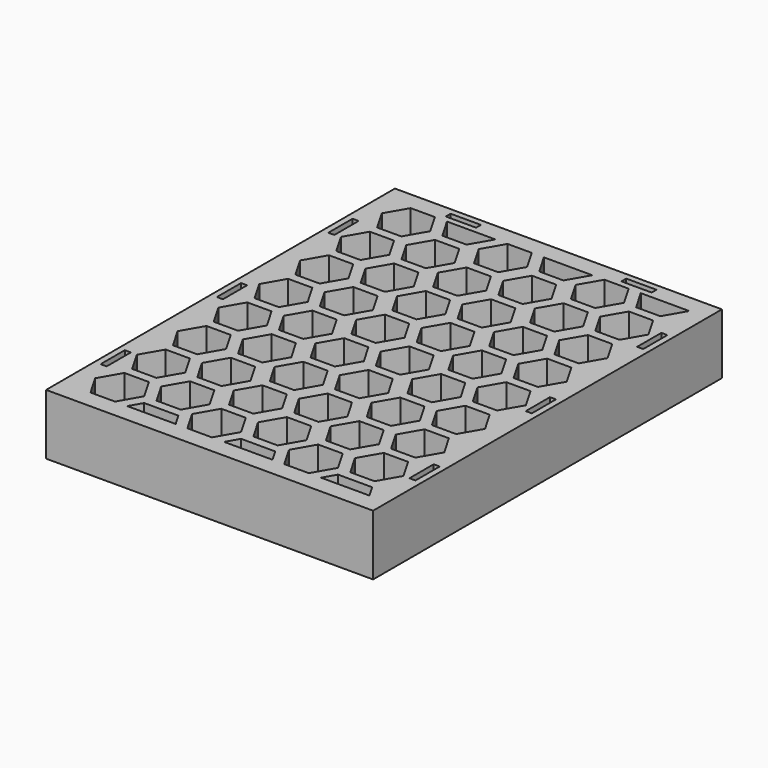
from build123d import *

# Parameters (mm, degrees)
F0_W     = 129.54
F0_H     = 179.07
F1_DEPTH = 25.4
F2_DEPTH = 25.4
F3_DEPTH = 25.4
F5_DEPTH = 25.4
F6_DEPTH = 25.4
F7_W     = 2.54
F7_H     = 12.7
F7_W_2   = 12.7
F7_H_2   = 2.54
F8_DEPTH = 7.62


# Not quite as in the source:
# - a feature names something its author has since deleted; it is built from what else it names


with BuildPart() as f1:
    # F0 (on Top) → F1 (new body)
    with BuildSketch(Plane.XY):
        with Locations((-8.2323685432, 21.6441547314)):
            Rectangle(F0_W, F0_H)
        Polygon((-69.4105034385, -51.3775724846), (-64.275970552, -42.4842987183), (-54.0069031043, -42.4842977514), (-48.8723685432, -51.3775705508), (-54.0069014297, -60.2708443171), (-64.2759688773, -60.270845284), align=None, mode=Mode.SUBTRACT)
        Polygon((-48.8723685432, -60.2708452686), (-45.8830056211, -55.0931168053), (-31.5417314652, -55.0931168053), (-28.5523685432, -60.2708452686), align=None, mode=Mode.SUBTRACT)
        Polygon((-28.7705034385, -51.3775720702), (-23.6359697633, -42.4842987593), (-13.3669023156, -42.4842987032), (-8.2323685432, -51.377571958), (-13.3669022184, -60.2708452689), (-23.635969666, -60.270845325), align=None, mode=Mode.SUBTRACT)
        Polygon((-48.8723685432, -42.4842987029), (-43.7923685432, -33.6854806004), (-33.6323685432, -33.6854806004), (-28.5523685432, -42.4842987029), (-33.6323685432, -51.2831168053), (-43.7923685432, -51.2831168053), align=None, mode=Mode.SUBTRACT)
        Polygon((-28.5523685432, -29.8754806837), (-23.4723685912, -21.0766625535), (-13.3123685912, -21.076662498), (-8.2323685432, -29.8754805727), (-13.3123684951, -38.6742987029), (-23.4723684951, -38.6742987584), align=None, mode=Mode.SUBTRACT)
        Polygon((-48.8723685432, -21.076662498), (-43.7923685432, -12.2778443955), (-33.6323685432, -12.2778443955), (-28.5523685432, -21.076662498), (-33.6323685432, -29.8754806004), (-43.7923685432, -29.8754806004), align=None, mode=Mode.SUBTRACT)
        Polygon((-48.8723685432, 0.3309737069), (-43.7923685432, 9.1297918094), (-33.6323685432, 9.1297918094), (-28.5523685432, 0.3309737069), (-33.6323685432, -8.4678443955), (-43.7923685432, -8.4678443955), align=None, mode=Mode.SUBTRACT)
        Polygon((-28.5523685432, -8.4678444788), (-23.4723685912, 0.3309736514), (-13.3123685912, 0.3309737069), (-8.2323685432, -8.4678443678), (-13.3123684951, -17.266662498), (-23.4723684951, -17.2666625535), align=None, mode=Mode.SUBTRACT)
        Polygon((-48.8723685432, 21.7386099118), (-43.7923685432, 30.5374280143), (-33.6323685432, 30.5374280143), (-28.5523685432, 21.7386099118), (-33.6323685432, 12.9397918094), (-43.7923685432, 12.9397918094), align=None, mode=Mode.SUBTRACT)
        Polygon((-28.5523685432, 12.9397917261), (-23.4723685912, 21.7386098563), (-13.3123685912, 21.7386099118), (-8.2323685432, 12.9397918371), (-13.3123684951, 4.1409737069), (-23.4723684951, 4.1409736514), align=None, mode=Mode.SUBTRACT)
        Polygon((-8.2323685432, -60.2708452686), (-5.2430056211, -55.0931168053), (9.0982685348, -55.0931168053), (12.0876314568, -60.2708452686), align=None, mode=Mode.SUBTRACT)
        Polygon((11.8694965615, -51.3775719857), (17.0040302854, -42.4842987029), (27.273097733, -42.4842987029), (32.4076314568, -51.3775719857), (27.273097733, -60.2708452686), (17.0040302854, -60.2708452686), align=None, mode=Mode.SUBTRACT)
        Polygon((-8.2323685432, -42.4842987029), (-3.1523685432, -33.6854806004), (7.0076314568, -33.6854806004), (12.0876314568, -42.4842987029), (7.0076314568, -51.2831168053), (-3.1523685432, -51.2831168053), align=None, mode=Mode.SUBTRACT)
        Polygon((12.0876314568, -29.8754806004), (17.1676314568, -21.076662498), (27.3276314568, -21.076662498), (32.4076314568, -29.8754806004), (27.3276314568, -38.6742987029), (17.1676314568, -38.6742987029), align=None, mode=Mode.SUBTRACT)
        Polygon((32.4076314568, -60.2708452686), (35.3969943789, -55.0931168053), (49.7382685348, -55.0931168053), (52.7276314568, -60.2708452686), align=None, mode=Mode.SUBTRACT)
        Polygon((-8.2323685432, -21.076662498), (-3.1523685432, -12.2778443955), (7.0076314568, -12.2778443955), (12.0876314568, -21.076662498), (7.0076314568, -29.8754806004), (-3.1523685432, -29.8754806004), align=None, mode=Mode.SUBTRACT)
        Polygon((-8.2323685432, 0.3309737069), (-3.1523685432, 9.1297918094), (7.0076314568, 9.1297918094), (12.0876314568, 0.3309737069), (7.0076314568, -8.4678443955), (-3.1523685432, -8.4678443955), align=None, mode=Mode.SUBTRACT)
        Polygon((12.0876314568, -8.4678443955), (17.1676314568, 0.3309737069), (27.3276314568, 0.3309737069), (32.4076314568, -8.4678443955), (27.3276314568, -17.266662498), (17.1676314568, -17.266662498), align=None, mode=Mode.SUBTRACT)
        Polygon((-8.2323685432, 21.7386099118), (-3.1523685432, 30.5374280143), (7.0076314568, 30.5374280143), (12.0876314568, 21.7386099118), (7.0076314568, 12.9397918094), (-3.1523685432, 12.9397918094), align=None, mode=Mode.SUBTRACT)
        Polygon((12.0876314568, 12.9397918094), (17.1676314568, 21.7386099118), (27.3276314568, 21.7386099118), (32.4076314568, 12.9397918094), (27.3276314568, 4.1409737069), (17.1676314568, 4.1409737069), align=None, mode=Mode.SUBTRACT)
        Polygon((-48.8723685432, 43.1462461167), (-43.7923685432, 51.9450642192), (-33.6323685432, 51.9450642192), (-28.5523685432, 43.1462461167), (-33.6323685432, 34.3474280143), (-43.7923685432, 34.3474280143), align=None, mode=Mode.SUBTRACT)
        Polygon((-28.5523685432, 34.347427931), (-23.4723685912, 43.1462460612), (-13.3123685912, 43.1462461167), (-8.2323685432, 34.347428042), (-13.3123684951, 25.5486099118), (-23.4723684951, 25.5486098563), align=None, mode=Mode.SUBTRACT)
        Polygon((-48.8723685432, 64.5538823216), (-43.7923685432, 73.3527004241), (-33.6323685432, 73.3527004241), (-28.5523685432, 64.5538823216), (-33.6323685432, 55.7550642192), (-43.7923685432, 55.7550642192), align=None, mode=Mode.SUBTRACT)
        Polygon((-28.5523685432, 55.7550641359), (-23.4723685912, 64.5538822661), (-13.3123685912, 64.5538823216), (-8.2323685432, 55.7550642469), (-13.3123684951, 46.9562461167), (-23.4723684951, 46.9562460612), align=None, mode=Mode.SUBTRACT)
        Polygon((-69.1923685432, 98.5703361507), (-64.1123693716, 107.3691547314), (-53.9523693716, 107.369155688), (-48.8723685432, 98.5703380639), (-53.9523677147, 89.7715194831), (-64.1123677147, 89.7715185265), align=None, mode=Mode.SUBTRACT)
        Polygon((-48.8723685432, 85.9615185265), (-43.7923685432, 94.760336629), (-33.6323685432, 94.760336629), (-28.5523685432, 85.9615185265), (-33.6323685432, 77.1627004241), (-43.7923685432, 77.1627004241), align=None, mode=Mode.SUBTRACT)
        Polygon((-28.5523685432, 77.1627003408), (-23.4723685912, 85.961518471), (-13.3123685912, 85.9615185265), (-8.2323685432, 77.1627004518), (-13.3123684951, 68.3638823216), (-23.4723684951, 68.3638822661), align=None, mode=Mode.SUBTRACT)
        Polygon((-43.7923685432, 98.570336629), (-48.8723685432, 107.3691547314), (-28.5523685432, 107.3691547314), (-33.6323685432, 98.570336629), align=None, mode=Mode.SUBTRACT)
        Polygon((-28.5523685432, 98.5703365457), (-23.4723685912, 107.3691546759), (-13.3123685912, 107.3691547314), (-8.2323685432, 98.5703366567), (-13.3123684951, 89.7715185265), (-23.4723684951, 89.771518471), align=None, mode=Mode.SUBTRACT)
        Polygon((-8.2323685432, 43.1462461167), (-3.1523685432, 51.9450642192), (7.0076314568, 51.9450642192), (12.0876314568, 43.1462461167), (7.0076314568, 34.3474280143), (-3.1523685432, 34.3474280143), align=None, mode=Mode.SUBTRACT)
        Polygon((12.0876314568, 34.3474280143), (17.1676314568, 43.1462461167), (27.3276314568, 43.1462461167), (32.4076314568, 34.3474280143), (27.3276314568, 25.5486099118), (17.1676314568, 25.5486099118), align=None, mode=Mode.SUBTRACT)
        Polygon((-8.2323685432, 64.5538823216), (-3.1523685432, 73.3527004241), (7.0076314568, 73.3527004241), (12.0876314568, 64.5538823216), (7.0076314568, 55.7550642192), (-3.1523685432, 55.7550642192), align=None, mode=Mode.SUBTRACT)
        Polygon((12.0876314568, 55.7550642192), (17.1676314568, 64.5538823216), (27.3276314568, 64.5538823216), (32.4076314568, 55.7550642192), (27.3276314568, 46.9562461167), (17.1676314568, 46.9562461167), align=None, mode=Mode.SUBTRACT)
        Polygon((-8.2323685432, 85.9615185265), (-3.1523685432, 94.760336629), (7.0076314568, 94.760336629), (12.0876314568, 85.9615185265), (7.0076314568, 77.1627004241), (-3.1523685432, 77.1627004241), align=None, mode=Mode.SUBTRACT)
        Polygon((12.0876314568, 77.1627004241), (17.1676314568, 85.9615185265), (27.3276314568, 85.9615185265), (32.4076314568, 77.1627004241), (27.3276314568, 68.3638823216), (17.1676314568, 68.3638823216), align=None, mode=Mode.SUBTRACT)
        Polygon((-3.1523685432, 98.570336629), (-8.2323685432, 107.3691547314), (12.0876314568, 107.3691547314), (7.0076314568, 98.570336629), align=None, mode=Mode.SUBTRACT)
        Polygon((12.0876314568, 98.570336629), (17.1676314568, 107.3691547314), (27.3276314568, 107.3691547314), (32.4076314568, 98.570336629), (27.3276314568, 89.7715185265), (17.1676314568, 89.7715185265), align=None, mode=Mode.SUBTRACT)
        Polygon((37.4876314568, 98.570336629), (32.4076314568, 107.3691547314), (52.7276314568, 107.3691547314), (47.6476314568, 98.570336629), align=None, mode=Mode.SUBTRACT)
        Polygon((27.273097733, -42.4842987029), (17.0040302854, -42.4842987029), (11.8694965615, -51.3775719857), (17.0040302854, -60.2708452686), (27.273097733, -60.2708452686), (32.4076314568, -51.3775719857), align=None)
        Polygon((-13.3669023156, -42.4842987032), (-23.6359697633, -42.4842987593), (-28.7705034385, -51.3775720702), (-23.635969666, -60.270845325), (-13.3669022184, -60.2708452689), (-8.2323685432, -51.377571958), align=None)
        Polygon((-54.0069031043, -42.4842977514), (-64.275970552, -42.4842987183), (-69.4105034385, -51.3775724846), (-64.2759688773, -60.270845284), (-54.0069014297, -60.2708443171), (-48.8723685432, -51.3775705508), align=None)
        Polygon((-33.6323685432, 51.9450642192), (-43.7923685432, 51.9450642192), (-48.8723685432, 43.1462461167), (-43.7923685432, 34.3474280143), (-33.6323685432, 34.3474280143), (-28.5523685432, 43.1462461167), align=None)
        Polygon((-13.3123685912, 43.1462461167), (-23.4723685912, 43.1462460612), (-28.5523685432, 34.347427931), (-23.4723684951, 25.5486098563), (-13.3123684951, 25.5486099118), (-8.2323685432, 34.347428042), align=None)
        Polygon((-13.3123685912, 21.7386099118), (-23.4723685912, 21.7386098563), (-28.5523685432, 12.9397917261), (-23.4723684951, 4.1409736514), (-13.3123684951, 4.1409737069), (-8.2323685432, 12.9397918371), align=None)
        Polygon((-13.3123685912, 0.3309737069), (-23.4723685912, 0.3309736514), (-28.5523685432, -8.4678444788), (-23.4723684951, -17.2666625535), (-13.3123684951, -17.266662498), (-8.2323685432, -8.4678443678), align=None)
        Polygon((-33.6323685432, -12.2778443955), (-43.7923685432, -12.2778443955), (-48.8723685432, -21.076662498), (-43.7923685432, -29.8754806004), (-33.6323685432, -29.8754806004), (-28.5523685432, -21.076662498), align=None)
        Polygon((-13.3123685912, -21.076662498), (-23.4723685912, -21.0766625535), (-28.5523685432, -29.8754806837), (-23.4723684951, -38.6742987584), (-13.3123684951, -38.6742987029), (-8.2323685432, -29.8754805727), align=None)
        Polygon((-33.6323685432, -33.6854806004), (-43.7923685432, -33.6854806004), (-48.8723685432, -42.4842987029), (-43.7923685432, -51.2831168053), (-33.6323685432, -51.2831168053), (-28.5523685432, -42.4842987029), align=None)
        Polygon((7.0076314568, -12.2778443955), (-3.1523685432, -12.2778443955), (-8.2323685432, -21.076662498), (-3.1523685432, -29.8754806004), (7.0076314568, -29.8754806004), (12.0876314568, -21.076662498), align=None)
        Polygon((7.0076314568, 9.1297918094), (-3.1523685432, 9.1297918094), (-8.2323685432, 0.3309737069), (-3.1523685432, -8.4678443955), (7.0076314568, -8.4678443955), (12.0876314568, 0.3309737069), align=None)
        Polygon((27.3276314568, 0.3309737069), (17.1676314568, 0.3309737069), (12.0876314568, -8.4678443955), (17.1676314568, -17.266662498), (27.3276314568, -17.266662498), (32.4076314568, -8.4678443955), align=None)
        Polygon((27.3276314568, -21.076662498), (17.1676314568, -21.076662498), (12.0876314568, -29.8754806004), (17.1676314568, -38.6742987029), (27.3276314568, -38.6742987029), (32.4076314568, -29.8754806004), align=None)
        Polygon((27.3276314568, 21.7386099118), (17.1676314568, 21.7386099118), (12.0876314568, 12.9397918094), (17.1676314568, 4.1409737069), (27.3276314568, 4.1409737069), (32.4076314568, 12.9397918094), align=None)
        Polygon((7.0076314568, 30.5374280143), (-3.1523685432, 30.5374280143), (-8.2323685432, 21.7386099118), (-3.1523685432, 12.9397918094), (7.0076314568, 12.9397918094), (12.0876314568, 21.7386099118), align=None)
        Polygon((27.3276314568, 43.1462461167), (17.1676314568, 43.1462461167), (12.0876314568, 34.3474280143), (17.1676314568, 25.5486099118), (27.3276314568, 25.5486099118), (32.4076314568, 34.3474280143), align=None)
        Polygon((7.0076314568, 51.9450642192), (-3.1523685432, 51.9450642192), (-8.2323685432, 43.1462461167), (-3.1523685432, 34.3474280143), (7.0076314568, 34.3474280143), (12.0876314568, 43.1462461167), align=None)
        Polygon((27.3276314568, 64.5538823216), (17.1676314568, 64.5538823216), (12.0876314568, 55.7550642192), (17.1676314568, 46.9562461167), (27.3276314568, 46.9562461167), (32.4076314568, 55.7550642192), align=None)
        Polygon((7.0076314568, 73.3527004241), (-3.1523685432, 73.3527004241), (-8.2323685432, 64.5538823216), (-3.1523685432, 55.7550642192), (7.0076314568, 55.7550642192), (12.0876314568, 64.5538823216), align=None)
        Polygon((-13.3123685912, 64.5538823216), (-23.4723685912, 64.5538822661), (-28.5523685432, 55.7550641359), (-23.4723684951, 46.9562460612), (-13.3123684951, 46.9562461167), (-8.2323685432, 55.7550642469), align=None)
        Polygon((-33.6323685432, 73.3527004241), (-43.7923685432, 73.3527004241), (-48.8723685432, 64.5538823216), (-43.7923685432, 55.7550642192), (-33.6323685432, 55.7550642192), (-28.5523685432, 64.5538823216), align=None)
        Polygon((-33.6323685432, 94.760336629), (-43.7923685432, 94.760336629), (-48.8723685432, 85.9615185265), (-43.7923685432, 77.1627004241), (-33.6323685432, 77.1627004241), (-28.5523685432, 85.9615185265), align=None)
        Polygon((-13.3123685912, 85.9615185265), (-23.4723685912, 85.961518471), (-28.5523685432, 77.1627003408), (-23.4723684951, 68.3638822661), (-13.3123684951, 68.3638823216), (-8.2323685432, 77.1627004518), align=None)
        Polygon((7.0076314568, 94.760336629), (-3.1523685432, 94.760336629), (-8.2323685432, 85.9615185265), (-3.1523685432, 77.1627004241), (7.0076314568, 77.1627004241), (12.0876314568, 85.9615185265), align=None)
        Polygon((27.3276314568, 85.9615185265), (17.1676314568, 85.9615185265), (12.0876314568, 77.1627004241), (17.1676314568, 68.3638823216), (27.3276314568, 68.3638823216), (32.4076314568, 77.1627004241), align=None)
        Polygon((7.0076314568, -33.6854806004), (-3.1523685432, -33.6854806004), (-8.2323685432, -42.4842987029), (-3.1523685432, -51.2831168053), (7.0076314568, -51.2831168053), (12.0876314568, -42.4842987029), align=None)
        Polygon((-53.9523693716, 107.369155688), (-64.1123693716, 107.3691547314), (-69.1923685432, 98.5703361507), (-64.1123677147, 89.7715185265), (-53.9523677147, 89.7715194831), (-48.8723685432, 98.5703380639), align=None)
        Polygon((27.3276314568, 107.3691547314), (17.1676314568, 107.3691547314), (12.0876314568, 98.570336629), (17.1676314568, 89.7715185265), (27.3276314568, 89.7715185265), (32.4076314568, 98.570336629), align=None)
        Polygon((-28.5523685432, 107.3691547314), (-48.8723685432, 107.3691547314), (-43.7923685432, 98.570336629), (-33.6323685432, 98.570336629), align=None)
        Polygon((52.7276314568, 107.3691547314), (32.4076314568, 107.3691547314), (37.4876314568, 98.570336629), (47.6476314568, 98.570336629), align=None)
        Polygon((49.7382685348, -55.0931168053), (35.3969943789, -55.0931168053), (32.4076314568, -60.2708452686), (52.7276314568, -60.2708452686), align=None)
        Polygon((9.0982685348, -55.0931168053), (-5.2430056211, -55.0931168053), (-8.2323685432, -60.2708452686), (12.0876314568, -60.2708452686), align=None)
        Polygon((-31.5417314652, -55.0931168053), (-45.8830056211, -55.0931168053), (-48.8723685432, -60.2708452686), (-28.5523685432, -60.2708452686), align=None)
    extrude(amount=F1_DEPTH)

    # F0 (on Top) → F2 (cut)
    with BuildSketch(Plane.XY):
        Polygon((-13.3123685912, -21.076662498), (-23.4723685912, -21.0766625535), (-28.5523685432, -29.8754806837), (-23.4723684951, -38.6742987584), (-13.3123684951, -38.6742987029), (-8.2323685432, -29.8754805727), align=None)
        Polygon((-33.6323685432, -12.2778443955), (-43.7923685432, -12.2778443955), (-48.8723685432, -21.076662498), (-43.7923685432, -29.8754806004), (-33.6323685432, -29.8754806004), (-28.5523685432, -21.076662498), align=None)
        Polygon((-33.6323685432, -33.6854806004), (-43.7923685432, -33.6854806004), (-48.8723685432, -42.4842987029), (-43.7923685432, -51.2831168053), (-33.6323685432, -51.2831168053), (-28.5523685432, -42.4842987029), align=None)
        Polygon((-13.3123685912, 0.3309737069), (-23.4723685912, 0.3309736514), (-28.5523685432, -8.4678444788), (-23.4723684951, -17.2666625535), (-13.3123684951, -17.266662498), (-8.2323685432, -8.4678443678), align=None)
        Polygon((-13.3123685912, 21.7386099118), (-23.4723685912, 21.7386098563), (-28.5523685432, 12.9397917261), (-23.4723684951, 4.1409736514), (-13.3123684951, 4.1409737069), (-8.2323685432, 12.9397918371), align=None)
        Polygon((-13.3123685912, 43.1462461167), (-23.4723685912, 43.1462460612), (-28.5523685432, 34.347427931), (-23.4723684951, 25.5486098563), (-13.3123684951, 25.5486099118), (-8.2323685432, 34.347428042), align=None)
        Polygon((-13.3123685912, 64.5538823216), (-23.4723685912, 64.5538822661), (-28.5523685432, 55.7550641359), (-23.4723684951, 46.9562460612), (-13.3123684951, 46.9562461167), (-8.2323685432, 55.7550642469), align=None)
        Polygon((-13.3123685912, 85.9615185265), (-23.4723685912, 85.961518471), (-28.5523685432, 77.1627003408), (-23.4723684951, 68.3638822661), (-13.3123684951, 68.3638823216), (-8.2323685432, 77.1627004518), align=None)
        Polygon((7.0076314568, 94.760336629), (-3.1523685432, 94.760336629), (-8.2323685432, 85.9615185265), (-3.1523685432, 77.1627004241), (7.0076314568, 77.1627004241), (12.0876314568, 85.9615185265), align=None)
        Polygon((7.0076314568, 73.3527004241), (-3.1523685432, 73.3527004241), (-8.2323685432, 64.5538823216), (-3.1523685432, 55.7550642192), (7.0076314568, 55.7550642192), (12.0876314568, 64.5538823216), align=None)
        Polygon((7.0076314568, 51.9450642192), (-3.1523685432, 51.9450642192), (-8.2323685432, 43.1462461167), (-3.1523685432, 34.3474280143), (7.0076314568, 34.3474280143), (12.0876314568, 43.1462461167), align=None)
        Polygon((7.0076314568, 30.5374280143), (-3.1523685432, 30.5374280143), (-8.2323685432, 21.7386099118), (-3.1523685432, 12.9397918094), (7.0076314568, 12.9397918094), (12.0876314568, 21.7386099118), align=None)
        Polygon((7.0076314568, 9.1297918094), (-3.1523685432, 9.1297918094), (-8.2323685432, 0.3309737069), (-3.1523685432, -8.4678443955), (7.0076314568, -8.4678443955), (12.0876314568, 0.3309737069), align=None)
        Polygon((7.0076314568, -12.2778443955), (-3.1523685432, -12.2778443955), (-8.2323685432, -21.076662498), (-3.1523685432, -29.8754806004), (7.0076314568, -29.8754806004), (12.0876314568, -21.076662498), align=None)
        Polygon((7.0076314568, -33.6854806004), (-3.1523685432, -33.6854806004), (-8.2323685432, -42.4842987029), (-3.1523685432, -51.2831168053), (7.0076314568, -51.2831168053), (12.0876314568, -42.4842987029), align=None)
        Polygon((27.3276314568, -21.076662498), (17.1676314568, -21.076662498), (12.0876314568, -29.8754806004), (17.1676314568, -38.6742987029), (27.3276314568, -38.6742987029), (32.4076314568, -29.8754806004), align=None)
        Polygon((27.3276314568, 0.3309737069), (17.1676314568, 0.3309737069), (12.0876314568, -8.4678443955), (17.1676314568, -17.266662498), (27.3276314568, -17.266662498), (32.4076314568, -8.4678443955), align=None)
        Polygon((27.3276314568, 21.7386099118), (17.1676314568, 21.7386099118), (12.0876314568, 12.9397918094), (17.1676314568, 4.1409737069), (27.3276314568, 4.1409737069), (32.4076314568, 12.9397918094), align=None)
        Polygon((27.3276314568, 43.1462461167), (17.1676314568, 43.1462461167), (12.0876314568, 34.3474280143), (17.1676314568, 25.5486099118), (27.3276314568, 25.5486099118), (32.4076314568, 34.3474280143), align=None)
        Polygon((27.3276314568, 64.5538823216), (17.1676314568, 64.5538823216), (12.0876314568, 55.7550642192), (17.1676314568, 46.9562461167), (27.3276314568, 46.9562461167), (32.4076314568, 55.7550642192), align=None)
        Polygon((27.3276314568, 85.9615185265), (17.1676314568, 85.9615185265), (12.0876314568, 77.1627004241), (17.1676314568, 68.3638823216), (27.3276314568, 68.3638823216), (32.4076314568, 77.1627004241), align=None)
        Polygon((-33.6323685432, 51.9450642192), (-43.7923685432, 51.9450642192), (-48.8723685432, 43.1462461167), (-43.7923685432, 34.3474280143), (-33.6323685432, 34.3474280143), (-28.5523685432, 43.1462461167), align=None)
        Polygon((-33.6323685432, 73.3527004241), (-43.7923685432, 73.3527004241), (-48.8723685432, 64.5538823216), (-43.7923685432, 55.7550642192), (-33.6323685432, 55.7550642192), (-28.5523685432, 64.5538823216), align=None)
        Polygon((-33.6323685432, 94.760336629), (-43.7923685432, 94.760336629), (-48.8723685432, 85.9615185265), (-43.7923685432, 77.1627004241), (-33.6323685432, 77.1627004241), (-28.5523685432, 85.9615185265), align=None)
    extrude(amount=F2_DEPTH, mode=Mode.SUBTRACT)

    # F0 (on Top) → F3 (cut)
    with BuildSketch(Plane.XY):
        Polygon((-31.5417314652, -55.0931168053), (-45.8830056211, -55.0931168053), (-48.8723685432, -60.2708452686), (-28.5523685432, -60.2708452686), align=None)
        Polygon((9.0982685348, -55.0931168053), (-5.2430056211, -55.0931168053), (-8.2323685432, -60.2708452686), (12.0876314568, -60.2708452686), align=None)
        Polygon((49.7382685348, -55.0931168053), (35.3969943789, -55.0931168053), (32.4076314568, -60.2708452686), (52.7276314568, -60.2708452686), align=None)
        Polygon((52.7276314568, 107.3691547314), (32.4076314568, 107.3691547314), (37.4876314568, 98.570336629), (47.6476314568, 98.570336629), align=None)
        Polygon((-28.5523685432, 107.3691547314), (-48.8723685432, 107.3691547314), (-43.7923685432, 98.570336629), (-33.6323685432, 98.570336629), align=None)
        Polygon((-13.3669023156, -42.4842987032), (-23.6359697633, -42.4842987593), (-28.7705034385, -51.3775720702), (-23.635969666, -60.270845325), (-13.3669022184, -60.2708452689), (-8.2323685432, -51.377571958), align=None)
        Polygon((27.273097733, -42.4842987029), (17.0040302854, -42.4842987029), (11.8694965615, -51.3775719857), (17.0040302854, -60.2708452686), (27.273097733, -60.2708452686), (32.4076314568, -51.3775719857), align=None)
        Polygon((27.3276314568, 107.3691547314), (17.1676314568, 107.3691547314), (12.0876314568, 98.570336629), (17.1676314568, 89.7715185265), (27.3276314568, 89.7715185265), (32.4076314568, 98.570336629), align=None)
        Polygon((-53.9523693716, 107.369155688), (-64.1123693716, 107.3691547314), (-69.1923685432, 98.5703361507), (-64.1123677147, 89.7715185265), (-53.9523677147, 89.7715194831), (-48.8723685432, 98.5703380639), align=None)
        Polygon((-54.0069031043, -42.4842977514), (-64.275970552, -42.4842987183), (-69.4105034385, -51.3775724846), (-64.2759688773, -60.270845284), (-54.0069014297, -60.2708443171), (-48.8723685432, -51.3775705508), align=None)
    extrude(amount=F3_DEPTH, mode=Mode.SUBTRACT)

    # F4 (on face) → F5 (cut)
    with BuildSketch(Plane.XY):
        Polygon((32.4076314568, -42.4842987029), (37.4876314568, -51.2831168053), (47.6476314568, -51.2831168053), (52.7276314568, -42.4842987029), (47.6476314568, -33.6854806004), (37.4876314568, -33.6854806004), align=None)
        Polygon((32.4076314568, -21.076662498), (37.4876314568, -29.8754806004), (47.6476314568, -29.8754806004), (52.7276314568, -21.076662498), (47.6476314568, -12.2778443955), (37.4876314568, -12.2778443955), align=None)
        Polygon((32.4076314568, 0.3309737069), (37.4876314568, -8.4678443955), (47.6476314568, -8.4678443955), (52.7276314568, 0.3309737069), (47.6476314568, 9.1297918094), (37.4876314568, 9.1297918094), align=None)
        Polygon((32.4076314568, 21.7386099118), (37.4876314568, 12.9397918094), (47.6476314568, 12.9397918094), (52.7276314568, 21.7386099118), (47.6476314568, 30.5374280143), (37.4876314568, 30.5374280143), align=None)
        Polygon((32.4076314568, 43.1462461167), (37.4876314568, 34.3474280143), (47.6476314568, 34.3474280143), (52.7276314568, 43.1462461167), (47.6476314568, 51.9450642192), (37.4876314568, 51.9450642192), align=None)
        Polygon((32.4076314568, 64.5538823216), (37.4876314568, 55.7550642192), (47.6476314568, 55.7550642192), (52.7276314568, 64.5538823216), (47.6476314568, 73.3527004241), (37.4876314568, 73.3527004241), align=None)
        Polygon((32.4076314568, 85.9615185265), (37.4876314568, 77.1627004241), (47.6476314568, 77.1627004241), (52.7276314568, 85.9615185265), (47.6476314568, 94.760336629), (37.4876314568, 94.760336629), align=None)
        Polygon((-69.1923685432, 77.1626999458), (-64.1123677147, 68.3638823216), (-53.9523677147, 68.3638832782), (-48.8723685432, 77.162701859), (-53.9523693716, 85.9615194831), (-64.1123693716, 85.9615185265), align=None)
        Polygon((-69.1923685432, 55.7550637409), (-64.1123677147, 46.9562461167), (-53.9523677147, 46.9562470733), (-48.8723685432, 55.7550656541), (-53.9523693716, 64.5538832782), (-64.1123693716, 64.5538823216), align=None)
        Polygon((-69.1923685432, 34.347427536), (-64.1123677147, 25.5486099118), (-53.9523677147, 25.5486108684), (-48.8723685432, 34.3474294492), (-53.9523693716, 43.1462470733), (-64.1123693716, 43.1462461167), align=None)
        Polygon((-69.1923685432, 12.9397913311), (-64.1123677147, 4.1409737069), (-53.9523677147, 4.1409746635), (-48.8723685432, 12.9397932443), (-53.9523693716, 21.7386108684), (-64.1123693716, 21.7386099118), align=None)
        Polygon((-69.1923685432, -8.4678448738), (-64.1123677147, -17.266662498), (-53.9523677147, -17.2666615414), (-48.8723685432, -8.4678429606), (-53.9523693716, 0.3309746635), (-64.1123693716, 0.3309737069), align=None)
        Polygon((-69.1923685432, -29.8754810787), (-64.1123677147, -38.6742987029), (-53.9523677147, -38.6742977463), (-48.8723685432, -29.8754791655), (-53.9523693716, -21.0766615414), (-64.1123693716, -21.076662498), align=None)
    extrude(amount=F5_DEPTH, mode=Mode.SUBTRACT)

    # F0 (on Top) → F6 (join)
    with BuildSketch(Plane.XY):
        Polygon((60.3476314568, 114.9891547314), (-76.8123685432, 114.9891547314), (-76.8123685432, -67.8908452686), (-73.0023685432, -67.8908452686), (-73.0023685432, 111.1791547314), (56.5376314568, 111.1791547314), (56.5376314568, -67.8908452686), (60.3476314568, -67.8908452686), align=None)
    extrude(amount=F6_DEPTH)

    # F7 (on face) → F8 (cut)
    with BuildSketch(Plane.XY.offset(25.4)):
        with Locations((-73.0023685432, -36.1408452686)):
            Rectangle(F7_W, F7_H)
        with Locations((-73.0023685432, 24.8191547314)):
            Rectangle(F7_W, F7_H)
        with Locations((56.5376314568, -36.1408452686)):
            Rectangle(F7_W, F7_H)
        with Locations((56.5376314568, 24.8191547314)):
            Rectangle(F7_W, F7_H)
        with Locations((-73.0023685432, 83.2391547314)):
            Rectangle(F7_W, F7_H)
        with Locations((56.5376314568, 83.2391547314)):
            Rectangle(F7_W, F7_H)
        with Locations((-45.0623685432, 111.1791547314)):
            Rectangle(F7_W_2, F7_H_2)
        with Locations((28.5976314568, 111.1791547314)):
            Rectangle(F7_W_2, F7_H_2)
    extrude(amount=-F8_DEPTH, mode=Mode.SUBTRACT)


solid = f1.part
